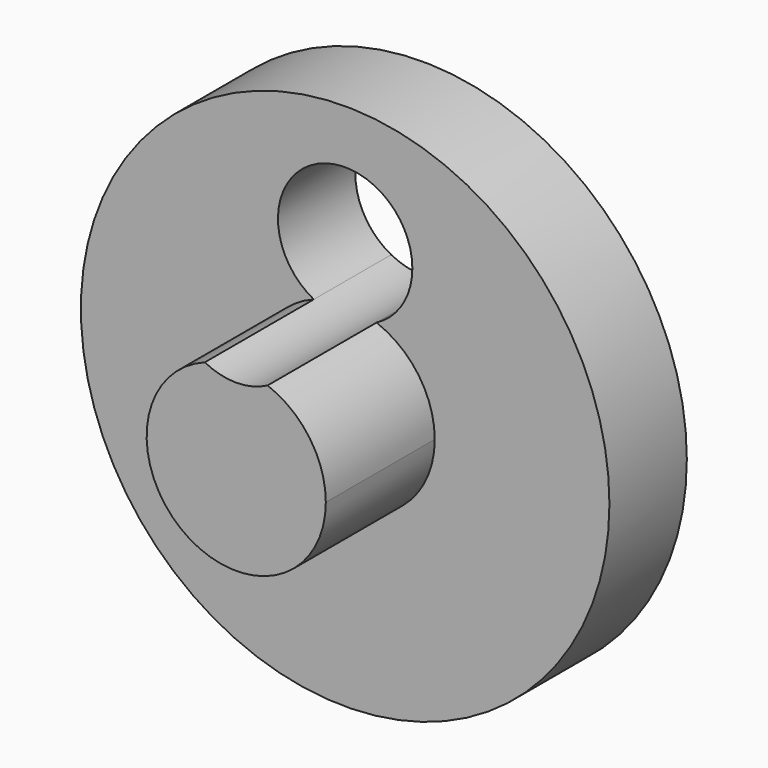
from build123d import *

# Parameters (mm, degrees)
F0_R     = 147.5
F1_DEPTH = 54
F2_DEPTH = 54
F3_DEPTH = 130


with BuildPart() as f1:
    # F0 (on Front) → F1 (new body)
    with BuildSketch(Plane.XZ):
        with Locations((-82.275771, -14.585894)):
            Circle(F0_R)
        with BuildLine():
            ThreePointArc((-64.771629, 32.250044), (-41.195319, 13.916676), (-32.275771, -14.585894))
            ThreePointArc((-32.275771, -14.585894), (-110.77834, -55.666346), (-99.779912, 32.250044))
            ThreePointArc((-99.779912, 32.250044), (-101.638682, 97.528397), (-44.775771, 65.414106))
            ThreePointArc((-44.775771, 65.414106), (-50.16148, 46.051195), (-64.771629, 32.250044))
        make_face(mode=Mode.SUBTRACT)
        with BuildLine():
            ThreePointArc((-99.779912, 32.250044), (-82.275771, 35.414106), (-64.771629, 32.250044))
            ThreePointArc((-64.771629, 32.250044), (-50.16148, 46.051195), (-44.775771, 65.414106))
            ThreePointArc((-44.775771, 65.414106), (-101.638682, 97.528397), (-99.779912, 32.250044))
        make_face()
        with BuildLine():
            ThreePointArc((-99.779912, 32.250044), (-110.77834, -55.666346), (-32.275771, -14.585894))
            ThreePointArc((-32.275771, -14.585894), (-41.195319, 13.916676), (-64.771629, 32.250044))
            ThreePointArc((-64.771629, 32.250044), (-82.275771, 27.914106), (-99.779912, 32.250044))
        make_face()
        with BuildLine():
            ThreePointArc((-99.779912, 32.250044), (-82.275771, 27.914106), (-64.771629, 32.250044))
            ThreePointArc((-64.771629, 32.250044), (-82.275771, 35.414106), (-99.779912, 32.250044))
        make_face()
    extrude(amount=F1_DEPTH)

    # F0 (on Front) → F2 (cut)
    with BuildSketch(Plane.XZ):
        with BuildLine():
            ThreePointArc((-99.779912, 32.250044), (-82.275771, 35.414106), (-64.771629, 32.250044))
            ThreePointArc((-64.771629, 32.250044), (-50.16148, 46.051195), (-44.775771, 65.414106))
            ThreePointArc((-44.775771, 65.414106), (-101.638682, 97.528397), (-99.779912, 32.250044))
        make_face()
        with BuildLine():
            ThreePointArc((-99.779912, 32.250044), (-82.275771, 27.914106), (-64.771629, 32.250044))
            ThreePointArc((-64.771629, 32.250044), (-82.275771, 35.414106), (-99.779912, 32.250044))
        make_face()
    extrude(amount=F2_DEPTH, mode=Mode.SUBTRACT)

    # F0 (on Front) → F3 (join)
    with BuildSketch(Plane.XZ):
        with BuildLine():
            ThreePointArc((-99.779912, 32.250044), (-110.77834, -55.666346), (-32.275771, -14.585894))
            ThreePointArc((-32.275771, -14.585894), (-41.195319, 13.916676), (-64.771629, 32.250044))
            ThreePointArc((-64.771629, 32.250044), (-82.275771, 27.914106), (-99.779912, 32.250044))
        make_face()
    extrude(amount=F3_DEPTH)


solid = f1.part
